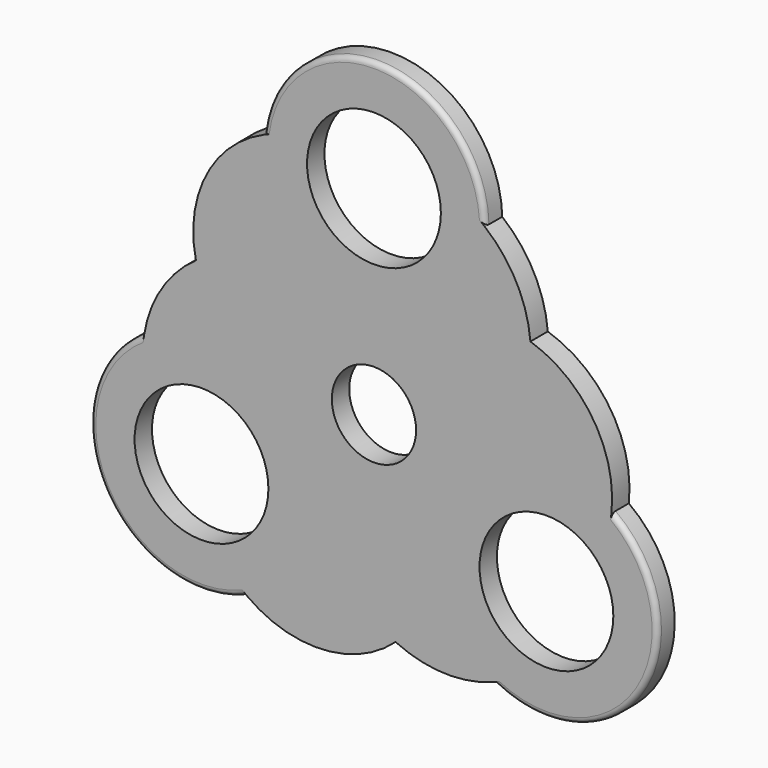
from build123d import *

# Parameters (mm, degrees)
F0_R         = 19.5450228134
F0_R_2       = 12.3084359059
F1_DEPTH     = 6.35
F2_T4_ANGLE  = 186.4329686672
F2_S5_R      = 36.413303104
F2_T6_DEPTH  = 41
F2_S7_R      = 34.3943026377
F2_T8_DEPTH  = 41
F2_T12_ANGLE = 186.4329686672
F2_S13_R     = 36.413303104
F2_T14_DEPTH = 44
F2_S15_R     = 34.3943026377
F2_T16_DEPTH = 44
F2_T20_ANGLE = 186.4329686672
F2_S21_R     = 36.413303104
F2_T22_DEPTH = 43
F2_S23_R     = 34.3943026377
F2_T24_DEPTH = 43


# Not quite as in the source:
# - a fillet or chamfer that OpenCascade refuses, or shapes differently, is made with other operations: its cross-section is extruded or revolved along the edge and cut away or added


with BuildPart() as f1:
    # F0 (on Front) → F1 (new body)
    with BuildSketch(Plane.XZ):
        with BuildLine():
            ThreePointArc((45.7058369334, 33.6726559303), (41.6121725533, 47.6126804082), (32.3941794324, 58.8425946254))
            ThreePointArc((32.3941794324, 58.8425946254), (1.3289124245, 90.5489995431), (-32.2304944376, 61.495374328))
            ThreePointArc((-32.2304944376, 61.495374328), (-49.0277697558, 45.6463332306), (-52.0142939153, 22.7460879204))
            ThreePointArc((-52.0142939153, 22.7460879204), (-62.0398770524, 12.2308583337), (-67.1562714864, -1.3671149894))
            ThreePointArc((-67.1562714864, -1.3671149894), (-79.0821901038, -44.1236278525), (-37.1413091645, -58.6601141235))
            ThreePointArc((-37.1413091645, -58.6601141235), (-15.0169992894, -65.2824607147), (6.3084569819, -56.4187438507))
            ThreePointArc((6.3084569819, -56.4187438507), (20.4277044991, -59.8435387419), (34.7620920539, -57.4754796359))
            ThreePointArc((34.7620920539, -57.4754796359), (77.7532776793, -46.4253716906), (69.3718036021, -2.8352602045))
            ThreePointArc((69.3718036021, -2.8352602045), (64.0447690452, 19.6361274841), (45.7058369334, 33.6726559303))
        make_face()
        with Locations((-50.3812096523, -29.0876049548)):
            Circle(F0_R, mode=Mode.SUBTRACT)
        with Locations((50.3812096523, -29.0876049548)):
            Circle(F0_R, mode=Mode.SUBTRACT)
        Circle(F0_R_2, mode=Mode.SUBTRACT)
        with Locations((0, 58.1752099097)):
            Circle(F0_R, mode=Mode.SUBTRACT)
    extrude(amount=F1_DEPTH)

    # F2: fillet of radius 1.524 on 3 edges, made by hand


with BuildPart() as f2_tool2:
    # F2_s3 → F2_t4 (revolve)
    with BuildSketch(Plane(origin=(5.6170399672, 0, 57.627710491), x_dir=(0, 1, 0), z_dir=(-0.0970114178, 0, -0.9952832686))):
        with BuildLine():
            ThreePointArc((-4.826, 26.7573938379), (-5.9036307345, 26.3110245724), (-6.35, 25.2333938379))
            Line((-6.35, 25.2333938379), (-6.35, 26.7573938379))
            Line((-6.35, 26.7573938379), (-4.826, 26.7573938379))
        make_face()
    revolve(axis=Axis((0, -6.35, 58.1752099097), (0, -1, 0)), revolution_arc=F2_T4_ANGLE)

    # F2_s5 → F2_t6 (cut, symmetric)
    with BuildSketch(Plane.XZ.offset(5.6)):
        with Locations((9.423343912, 30.5889336513)):
            Circle(F2_S5_R)
    extrude(amount=F2_T6_DEPTH, both=True, mode=Mode.SUBTRACT)

    # F2_s7 → F2_t8 (cut, symmetric)
    with BuildSketch(Plane.XZ.offset(5.6)):
        with Locations((-18.3950397685, 30.0065152183)):
            Circle(F2_S7_R)
    extrude(amount=F2_T8_DEPTH, both=True, mode=Mode.SUBTRACT)


with BuildPart() as f1_1:
    add(f1.part)

    # F2_t1: cut F2_tool2
    add(f2_tool2.part, mode=Mode.SUBTRACT)


with BuildPart() as f2_tool10:
    # F2_s11 → F2_t12 (revolve)
    with BuildSketch(Plane(origin=(47.0985412635, 0, -33.6783545512), x_dir=(0, 1, 0), z_dir=(-0.8134348857, 0, 0.5816559866))):
        with BuildLine():
            ThreePointArc((-4.826, 26.7573938379), (-5.9036307345, 26.3110245724), (-6.35, 25.2333938379))
            Line((-6.35, 25.2333938379), (-6.35, 26.7573938379))
            Line((-6.35, 26.7573938379), (-4.826, 26.7573938379))
        make_face()
    revolve(axis=Axis((50.3812096523, -6.35, -29.0876049548), (0, -1, 0)), revolution_arc=F2_T12_ANGLE)

    # F2_s13 → F2_t14 (cut, symmetric)
    with BuildSketch(Plane.XZ.offset(5.6)):
        with Locations((21.7791216607, -23.4553220421)):
            Circle(F2_S13_R)
    extrude(amount=F2_T14_DEPTH, both=True, mode=Mode.SUBTRACT)

    # F2_s15 → F2_t16 (cut, symmetric)
    with BuildSketch(Plane.XZ.offset(5.6)):
        with Locations((35.1839243423, 0.927314134)):
            Circle(F2_S15_R)
    extrude(amount=F2_T16_DEPTH, both=True, mode=Mode.SUBTRACT)


with BuildPart() as f1_2:
    add(f1_1.part)

    # F2_t9: cut F2_tool10
    add(f2_tool10.part, mode=Mode.SUBTRACT)


with BuildPart() as f2_tool18:
    # F2_s19 → F2_t20 (revolve)
    with BuildSketch(Plane(origin=(-52.7155812308, 0, -23.9493559398), x_dir=(0, 1, 0), z_dir=(0.9104463035, 0, 0.4136272821))):
        with BuildLine():
            ThreePointArc((-4.826, 26.7573938379), (-5.9036307345, 26.3110245724), (-6.35, 25.2333938379))
            Line((-6.35, 25.2333938379), (-6.35, 26.7573938379))
            Line((-6.35, 26.7573938379), (-4.826, 26.7573938379))
        make_face()
    revolve(axis=Axis((-50.3812096523, -6.35, -29.0876049548), (0, -1, 0)), revolution_arc=F2_T20_ANGLE)

    # F2_s21 → F2_t22 (cut, symmetric)
    with BuildSketch(Plane.XZ.offset(5.6)):
        with Locations((-31.2024655727, -7.1336116092)):
            Circle(F2_S21_R)
    extrude(amount=F2_T22_DEPTH, both=True, mode=Mode.SUBTRACT)

    # F2_s23 → F2_t24 (cut, symmetric)
    with BuildSketch(Plane.XZ.offset(5.6)):
        with Locations((-16.7888845738, -30.9338293523)):
            Circle(F2_S23_R)
    extrude(amount=F2_T24_DEPTH, both=True, mode=Mode.SUBTRACT)


with BuildPart() as f1_3:
    add(f1_2.part)

    # F2_t17: cut F2_tool18
    add(f2_tool18.part, mode=Mode.SUBTRACT)


solid = f1_3.part
